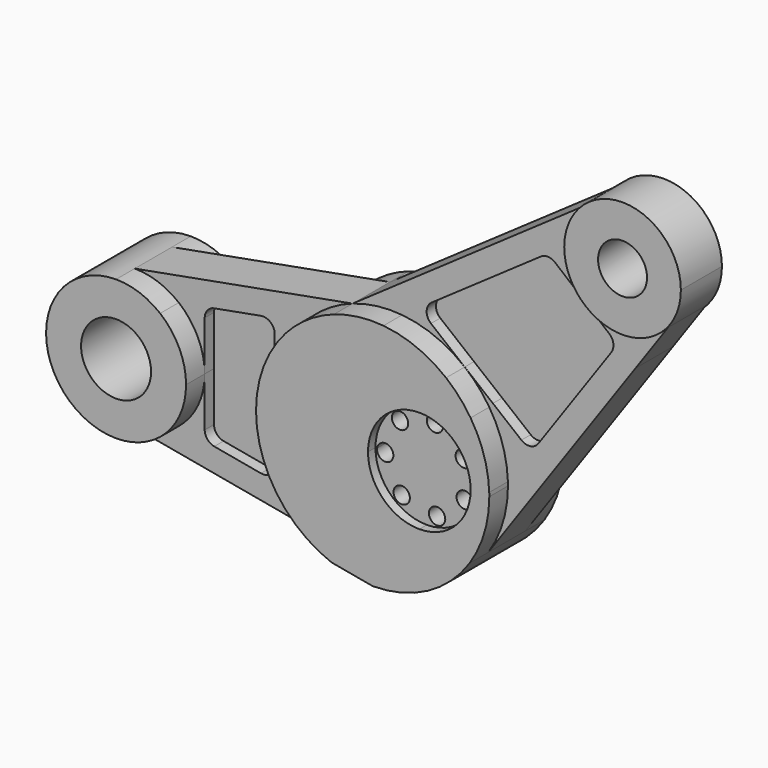
from build123d import *

# Parameters (mm, degrees)
F0_R     = 15
F1_DEPTH = 20
F2_DEPTH = 10
F3_DEPTH = 11
F0_R_2   = 3.5
F4_DEPTH = 16
F5_R     = 5
F5_2_R   = 5
F5_3_R   = 5
F5_4_R   = 5
F6_DEPTH = 5


# Not quite as in the source:
# - a feature names something its author has since deleted; it is built from what else it names


with BuildPart() as f1:
    # F0 (on Front) → F1 (new body, symmetric)
    with BuildSketch(Plane.XZ):
        with BuildLine():
            ThreePointArc((-111.07441, -23.277071), (-102.909709, -12.888605), (-100, 0))
            ThreePointArc((-100, 0), (-102.918839, 12.907778), (-111.107382, 23.30384))
            ThreePointArc((-111.107382, 23.30384), (-119.977905, 28.27645), (-130, 30))
            ThreePointArc((-130, 30), (-160, 0), (-130, -30))
            ThreePointArc((-130, -30), (-119.957892, -28.269349), (-111.07441, -23.277071))
        make_face()
        with Locations((-130, 0)):
            Circle(F0_R, mode=Mode.SUBTRACT)
    extrude(amount=F1_DEPTH, both=True)


with BuildPart() as f1b:
    # F0 (on Front) → F1, piece 2 (new body, symmetric)
    with BuildSketch(Plane.XZ):
        with BuildLine():
            ThreePointArc((-57.413965, 33.169191), (-66.747718, 17.738401), (-70, 0))
            Line((-70, 0), (-22, 0))
            ThreePointArc((-22, 0), (-15.556349, 15.556349), (0, 22))
            ThreePointArc((0, 22), (7.343751, 20.738113), (13.845049, 17.097211))
            Line((13.845049, 17.097211), (21.986192, 27.150685))
            ThreePointArc((21.986192, 27.150685), (17.189622, 33.420532), (11.466019, 38.857298))
            ThreePointArc((11.466019, 38.857298), (-1.132479, 46.303528), (-15.347309, 49.783054))
            ThreePointArc((-15.347309, 49.783054), (-26.125305, 49.623388), (-36.61862, 47.157412))
            ThreePointArc((-36.61862, 47.157412), (-47.906946, 41.487376), (-57.413965, 33.169191))
        make_face()
        with BuildLine():
            Line((-22, 0), (-70, 0))
            ThreePointArc((-70, 0), (-66.785848, -17.637587), (-57.556621, -33.007578))
            ThreePointArc((-57.556621, -33.007578), (-48.427468, -41.132458), (-37.6, -46.8))
            Line((-37.6, -46.8), (-20, -50))
            ThreePointArc((-20, -50), (3.568753, -44.096643), (21.572115, -27.780555))
            ThreePointArc((21.572115, -27.780555), (27.84666, -14.51541), (30, 0))
            ThreePointArc((30, 0), (29.99345, 0.809292), (29.973802, 1.618371))
            ThreePointArc((29.973802, 1.618371), (27.719334, 14.928668), (21.986192, 27.150685))
            Line((21.986192, 27.150685), (13.845049, 17.097211))
            ThreePointArc((13.845049, 17.097211), (19.856876, 9.471244), (22, 0))
            ThreePointArc((22, 0), (15.556349, -15.556349), (0, -22))
            ThreePointArc((0, -22), (-15.556349, -15.556349), (-22, 0))
        make_face()
    extrude(amount=F1_DEPTH, both=True)

    # F0 (on Front) → F4 (join, symmetric)
    with BuildSketch(Plane.XZ):
        with BuildLine():
            Line((-21.291582, 0), (-22, 0))
            ThreePointArc((-22, 0), (-15.556349, -15.556349), (0, -22))
            Line((0, -22), (0, 0))
            Line((0, 0), (-14.354289, 0))
            ThreePointArc((-14.354289, 0), (-14.330783, -0.23319), (-14.322936, -0.46743))
            ThreePointArc((-14.322936, -0.46743), (-18.057176, -3.959583), (-21.291582, 0))
        make_face()
        with Locations((-10.746967, -14.22597)):
            Circle(F0_R_2, mode=Mode.SUBTRACT)
        with BuildLine():
            ThreePointArc((0, 22), (-15.556349, 15.556349), (-22, 0))
            Line((-22, 0), (-21.291582, 0))
            ThreePointArc((-21.291582, 0), (-17.822936, 3.03257), (-14.354289, 0))
            Line((-14.354289, 0), (0, 0))
            Line((0, 0), (0, 22))
        make_face()
        with Locations((-11.47787, 13.643094)):
            Circle(F0_R_2, mode=Mode.SUBTRACT)
        with BuildLine():
            ThreePointArc((13.845049, 17.097211), (7.343751, 20.738113), (0, 22))
            Line((0, 22), (0, 0))
            Line((0, 0), (13.845049, 17.097211))
        make_face()
        with Locations((3.510266, 17.48009)):
            Circle(F0_R_2, mode=Mode.SUBTRACT)
        with BuildLine():
            Line((0, 0), (0, -22))
            ThreePointArc((0, -22), (15.556349, -15.556349), (22, 0))
            ThreePointArc((22, 0), (19.856876, 9.471244), (13.845049, 17.097211))
            Line((13.845049, 17.097211), (0, 0))
        make_face()
        with Locations((4.421687, -17.272064)):
            Circle(F0_R_2, mode=Mode.SUBTRACT)
        with Locations((16.26072, -7.311942)):
            Circle(F0_R_2, mode=Mode.SUBTRACT)
        with Locations((15.8551, 8.154222)):
            Circle(F0_R_2, mode=Mode.SUBTRACT)
    extrude(amount=F4_DEPTH, both=True)


with BuildPart() as f2:
    # F0 (on Front) → F2 (new body, symmetric)
    with BuildSketch(Plane.XZ):
        with BuildLine():
            ThreePointArc((-130, 30), (-119.977905, 28.27645), (-111.107382, 23.30384))
            Line((-111.107382, 23.30384), (-111.074099, 23.309956))
            Line((-111.074099, 23.309956), (-100, 25.344653))
            Line((-100, 25.344653), (-70, 30.856698))
            Line((-70, 30.856698), (-57.413965, 33.169191))
            ThreePointArc((-57.413965, 33.169191), (-47.906946, 41.487376), (-36.61862, 47.157412))
            Line((-36.61862, 47.157412), (-130, 30))
        make_face()
        with BuildLine():
            ThreePointArc((-111.107382, 23.30384), (-102.918839, 12.907778), (-100, 0))
            Line((-100, 0), (-100, 25.344653))
            Line((-100, 25.344653), (-111.074099, 23.309956))
            Line((-111.074099, 23.309956), (-111.107382, 23.30384))
        make_face()
        with BuildLine():
            Line((-70, 30.856698), (-70, 0))
            ThreePointArc((-70, 0), (-66.747718, 17.738401), (-57.413965, 33.169191))
            Line((-57.413965, 33.169191), (-70, 30.856698))
        make_face()
    extrude(amount=F2_DEPTH, both=True)

    # F5#2
    f5_2_edges = [f2.edges().sort_by_distance(p)[0] for p in [
        (-100, 0, 25.344653),
        (-70, 0, 30.856698),
    ]]
    fillet(f5_2_edges, radius=F5_2_R)


with BuildPart() as f2b:
    # F0 (on Front) → F2, piece 2 (new body, symmetric)
    with BuildSketch(Plane.XZ):
        with BuildLine():
            Line((-100, -25.2906), (-111.07441, -23.277071))
            ThreePointArc((-111.07441, -23.277071), (-119.957892, -28.269349), (-130, -30))
            Line((-130, -30), (-37.6, -46.8))
            ThreePointArc((-37.6, -46.8), (-48.427468, -41.132458), (-57.556621, -33.007578))
            Line((-57.556621, -33.007578), (-70, -30.745146))
            Line((-70, -30.745146), (-100, -25.2906))
        make_face()
        with BuildLine():
            Line((-100, -25.2906), (-100, 0))
            ThreePointArc((-100, 0), (-102.909709, -12.888605), (-111.07441, -23.277071))
            Line((-111.07441, -23.277071), (-100, -25.2906))
        make_face()
        with BuildLine():
            ThreePointArc((-57.556621, -33.007578), (-66.785848, -17.637587), (-70, 0))
            Line((-70, 0), (-70, -30.745146))
            Line((-70, -30.745146), (-57.556621, -33.007578))
        make_face()
    extrude(amount=F2_DEPTH, both=True)

    # F5
    f5_edges = [f2b.edges().sort_by_distance(p)[0] for p in [
        (-100, 0, -25.2906),
        (-70, 0, -30.745146),
    ]]
    fillet(f5_edges, radius=F5_R)


with BuildPart() as f2c:
    # F0 (on Front) → F2, piece 3 (new body, symmetric)
    with BuildSketch(Plane.XZ):
        with BuildLine():
            Line((84.678416, 62.213764), (98.638111, 82.121337))
            ThreePointArc((98.638111, 82.121337), (90.457485, 76.025105), (80.522573, 73.704711))
            Line((80.522573, 73.704711), (76.966056, 68.63285))
            Line((76.966056, 68.63285), (84.678416, 62.213764))
        make_face()
        with BuildLine():
            ThreePointArc((30, 0), (27.84666, -14.51541), (21.572115, -27.780555))
            Line((21.572115, -27.780555), (84.678416, 62.213764))
            Line((84.678416, 62.213764), (76.966056, 68.63285))
            Line((76.966056, 68.63285), (39.925959, 15.810894))
            Line((39.925959, 15.810894), (29.973802, 1.618371))
            ThreePointArc((29.973802, 1.618371), (29.99345, 0.809292), (30, 0))
        make_face()
        with BuildLine():
            Line((64.19068, 79.268888), (64.189255, 79.267129))
            Line((64.189255, 79.267129), (76.966056, 68.63285))
            Line((76.966056, 68.63285), (80.522573, 73.704711))
            ThreePointArc((80.522573, 73.704711), (71.861403, 75.033228), (64.19068, 79.268888))
        make_face()
        with BuildLine():
            Line((23.545136, 29.075822), (21.986192, 27.150685))
            ThreePointArc((21.986192, 27.150685), (27.719334, 14.928668), (29.973802, 1.618371))
            Line((29.973802, 1.618371), (39.925959, 15.810894))
            Line((39.925959, 15.810894), (23.545136, 29.075822))
        make_face()
        with BuildLine():
            ThreePointArc((11.466019, 38.857298), (17.189622, 33.420532), (21.986192, 27.150685))
            Line((21.986192, 27.150685), (23.545136, 29.075822))
            Line((23.545136, 29.075822), (11.466019, 38.857298))
        make_face()
    extrude(amount=F2_DEPTH, both=True)

    # F5#3
    f5_3_edges = [f2c.edges().sort_by_distance(p)[0] for p in [
        (76.966056, 0, 68.63285),
        (39.925959, 0, 15.810894),
    ]]
    fillet(f5_3_edges, radius=F5_3_R)


with BuildPart() as f2d:
    # F0 (on Front) → F2, piece 4 (new body, symmetric)
    with BuildSketch(Plane.XZ):
        with BuildLine():
            Line((61.209268, 115.273737), (-36.61862, 47.157412))
            ThreePointArc((-36.61862, 47.157412), (-26.125305, 49.623388), (-15.347309, 49.783054))
            Line((-15.347309, 49.783054), (-8.184801, 54.770219))
            Line((-8.184801, 54.770219), (47.2481, 93.367449))
            Line((47.2481, 93.367449), (54.923694, 98.711868))
            ThreePointArc((54.923694, 98.711868), (56.550383, 107.568193), (61.209268, 115.273737))
        make_face()
        with BuildLine():
            ThreePointArc((63.93067, 79.482352), (57.284114, 88.093311), (54.923694, 98.711868))
            Line((54.923694, 98.711868), (47.2481, 93.367449))
            Line((47.2481, 93.367449), (63.93067, 79.482352))
        make_face()
        with BuildLine():
            Line((-8.184801, 54.770219), (-15.347309, 49.783054))
            ThreePointArc((-15.347309, 49.783054), (-1.132479, 46.303528), (11.466019, 38.857298))
            Line((11.466019, 38.857298), (-8.184801, 54.770219))
        make_face()
    extrude(amount=F2_DEPTH, both=True)

    # F5#4
    f5_4_edges = [f2d.edges().sort_by_distance(p)[0] for p in [
        (47.2481, 0, 93.367449),
        (-8.184801, 0, 54.770219),
    ]]
    fillet(f5_4_edges, radius=F5_4_R)


with BuildPart() as f3:
    # F0 (on Front) → F3 (new body, symmetric)
    with BuildSketch(Plane.XZ):
        with BuildLine():
            ThreePointArc((104.92369, 98.697537), (88.787646, 122.073385), (61.209268, 115.273737))
            ThreePointArc((61.209268, 115.273737), (56.550383, 107.568193), (54.923694, 98.711868))
            ThreePointArc((54.923694, 98.711868), (57.284114, 88.093311), (63.93067, 79.482352))
            ThreePointArc((63.93067, 79.482352), (64.060316, 79.375183), (64.19068, 79.268888))
            ThreePointArc((64.19068, 79.268888), (71.861403, 75.033228), (80.522573, 73.704711))
            ThreePointArc((80.522573, 73.704711), (90.457485, 76.025105), (98.638111, 82.121337))
            ThreePointArc((98.638111, 82.121337), (103.299538, 89.83358), (104.92369, 98.697537))
        make_face()
        with BuildLine():
            ThreePointArc((90.42369, 98.697537), (84.444056, 89.220392), (73.315826, 90.537505))
            ThreePointArc((73.315826, 90.537505), (75.403323, 108.174683), (90.42369, 98.697537))
        make_face(mode=Mode.SUBTRACT)
    extrude(amount=F3_DEPTH, both=True)


with BuildPart() as f6:
    # F0 (on Front) → F6 (new body, symmetric)
    with BuildSketch(Plane.XZ):
        Polygon((-100, 25.344653), (-100, 0), (-70, 0), (-70, 30.856698), align=None)
        Polygon((-70, 0), (-100, 0), (-100, -25.2906), (-70, -30.745146), align=None)
    extrude(amount=F6_DEPTH, both=True)


with BuildPart() as f6b:
    # F0 (on Front) → F6, piece 2 (new body, symmetric)
    with BuildSketch(Plane.XZ):
        Polygon((-8.184801, 54.770219), (11.466019, 38.857298), (23.545136, 29.075822), (64.189255, 79.267129), (63.93067, 79.482352), (47.2481, 93.367449), align=None)
        Polygon((64.189255, 79.267129), (23.545136, 29.075822), (39.925959, 15.810894), (76.966056, 68.63285), align=None)
    extrude(amount=F6_DEPTH, both=True)


solid = Compound([f1.part, f1b.part, f2.part, f2b.part, f2c.part, f2d.part, f3.part, f6.part, f6b.part])
